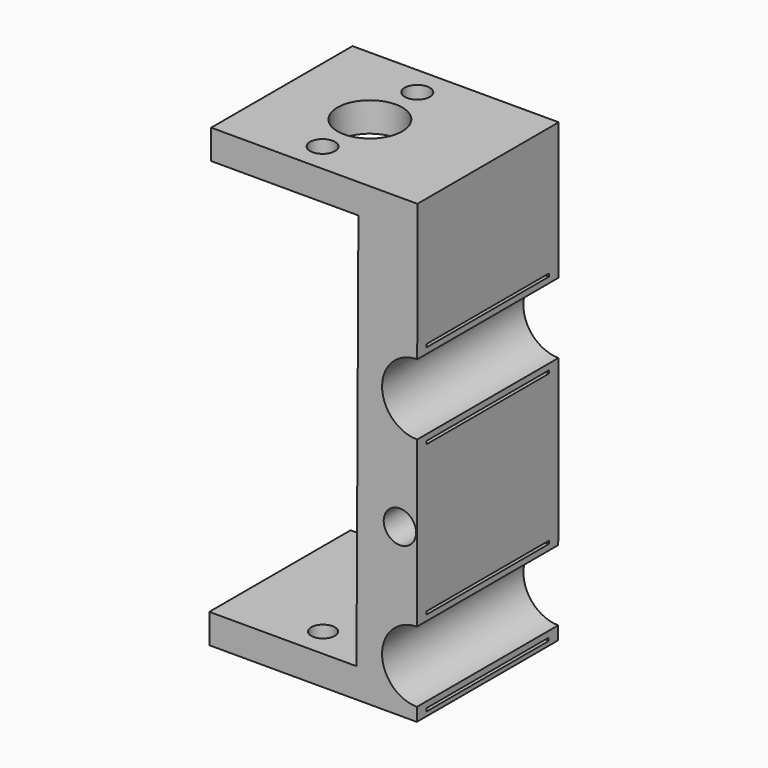
from build123d import *

# Parameters (mm, degrees)
F0_R           = 5.5
F1_DEPTH       = 60
F4_DEPTH       = 26
F4_DEPTH_BACK  = 26
F5_R           = 4
F6_DEPTH       = 5
F7_R           = 4.25
F8_DEPTH       = 15
F9_R           = 11
F10_DEPTH      = 25
F10_DEPTH_BACK = 25


# Not quite as in the source:
# - a feature names something its author has since deleted; it is built from what else it names


with BuildPart() as f1:
    # F0 (on Front) → F1 (new body)
    with BuildSketch(Plane.XZ):
        with BuildLine():
            ThreePointArc((-0.0872969156, -53.4805140133), (-11.9999962709, -41.4659778258), (-0.0575900904, -29.4809696761))
            Line((-0.0575900904, -29.4809696761), (-5.4639e-06, 17.0404876904))
            Line((-5.4639e-06, 17.0404876904), (-70.0428405992, 17.0404876904))
            Line((-70.0428405992, 17.0404876904), (-70.0428405992, 7.0404876904))
            Line((-70.0428405992, 7.0404876904), (-20.0428405992, 7.0404876904))
            Line((-20.0428405992, 7.0404876904), (-20.6929361639, -127.9595123096))
            Line((-20.6929361639, -127.9595123096), (-70.6929361639, -127.9595123096))
            Line((-70.6929361639, -127.9595123096), (-70.6929361639, -137.9595123096))
            Line((-70.6929361639, -137.9595123096), (-0.1918656855, -137.9595123096))
            Line((-0.1918656855, -137.9595123096), (-0.1862936956, -133.4580141387))
            ThreePointArc((-0.1862936956, -133.4580141387), (-11.9988136294, -121.4446249335), (-0.1565894029, -109.4605157571))
            Line((-0.1565894029, -109.4605157571), (-0.0872969156, -53.4805140133))
        make_face()
        with Locations((-5.947382655, -81.4808309078)):
            Circle(F0_R, mode=Mode.SUBTRACT)
    extrude(amount=F1_DEPTH)


with BuildPart() as f1_1:
    # F2: moved
    add(f1.part.moved(Location((0, 30, 0))))

    # F3 (on Front) → F4 (cut, two sides)
    with BuildSketch(Plane.XZ) as f4_sk:
        with BuildLine():
            ThreePointArc((0, -55.5154254436), (-14, -41.5154254436), (0, -27.5154254436))
            Line((0, -27.5154254436), (0, -26.5154254436))
            ThreePointArc((0, -26.5154254436), (-15, -41.5154254436), (0, -56.5154254436))
            Line((0, -56.5154254436), (0, -55.5154254436))
        make_face()
        with BuildLine():
            Line((0, -107.5154236555), (0, -106.5154236555))
            ThreePointArc((0, -106.5154236555), (-15, -121.5154236555), (0, -136.5154236555))
            Line((0, -136.5154236555), (0, -135.5154236555))
            ThreePointArc((0, -135.5154236555), (-14, -121.5154236555), (0, -107.5154236555))
        make_face()
    extrude(amount=F4_DEPTH, mode=Mode.SUBTRACT)
    extrude(f4_sk.sketch, amount=-F4_DEPTH_BACK, mode=Mode.SUBTRACT)

    # F5 (on face) → F6 (cut)
    with BuildSketch(Plane.XY.offset(-127.9595123096)):
        with Locations((-40.0428405992, -20)):
            Circle(F5_R)
        with Locations((-40.0428405992, 20)):
            Circle(F5_R)
    extrude(amount=-F6_DEPTH, mode=Mode.SUBTRACT)

    # F7 (on face) → F8 (cut)
    with BuildSketch(Plane.XY.offset(17.0404876904)):
        with Locations((-40.0428405992, 20)):
            Circle(F7_R)
        with Locations((-40.2286797762, -20)):
            Circle(F7_R)
    extrude(amount=-F8_DEPTH, mode=Mode.SUBTRACT)

    # F9 (on face) → F10 (cut, two sides)
    with BuildSketch(Plane.XY.offset(17.0404876904)) as f10_sk:
        with Locations((-40.1357601877, 0)):
            Circle(F9_R)
    extrude(amount=-F10_DEPTH, mode=Mode.SUBTRACT)
    extrude(f10_sk.sketch, amount=F10_DEPTH_BACK, mode=Mode.SUBTRACT)


solid = f1_1.part
